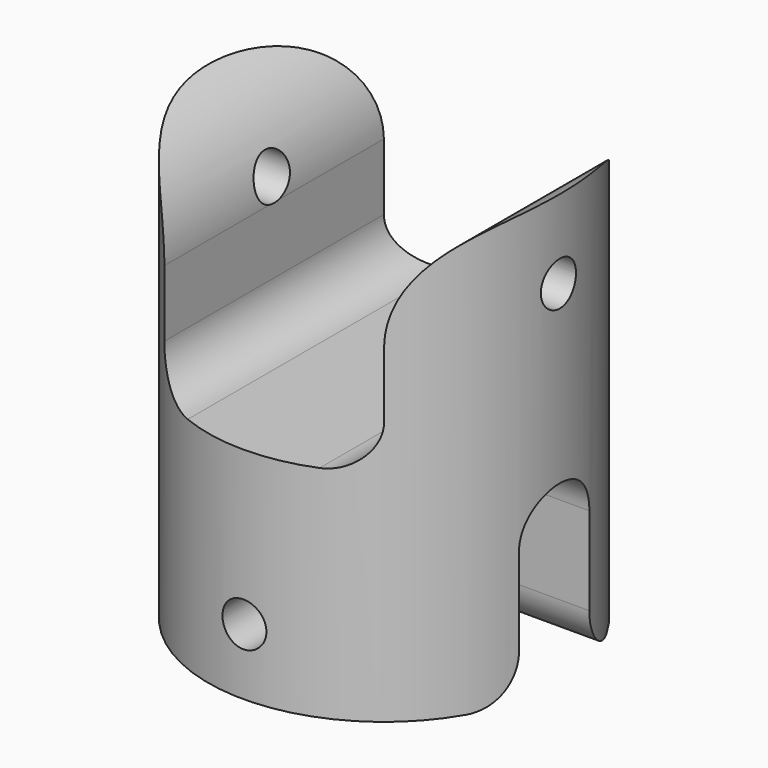
from build123d import *

# Parameters (mm, degrees)
F0_R         = 8
F1_DEPTH     = 20
F3_DEPTH     = 10
F5_DEPTH     = 8
F7_D         = 2
F7_DEPTH     = 3.001
F9_D         = 2
F10_T1_DEPTH = 37.4894960018
F12_D        = 2
F12_DEPTH    = 6.0010001
F14_D        = 2
F15_R        = 2
F16_R        = 1.9999


# Not quite as in the source:
# - a fillet or chamfer that OpenCascade refuses, or shapes differently, is made with other operations: its cross-section is extruded or revolved along the edge and cut away or added
# - a fillet or chamfer is up to 0.001 mm smaller than in the source, because OpenCascade refuses the exact size


with BuildPart() as f1:
    # F0 (on Top) → F1 (new body)
    with BuildSketch(Plane.XY):
        Circle(F0_R)
    extrude(amount=F1_DEPTH)

    # F2 (on face) → F3 (cut)
    with BuildSketch(Plane.XY.offset(20)):
        with BuildLine():
            ThreePointArc((5, 6.2449979984), (0, 8), (-5, 6.2449979984))
            Line((-5, 6.2449979984), (-5, -6.2449979984))
            ThreePointArc((-5, -6.2449979984), (0, -8), (5, -6.2449979984))
            Line((5, -6.2449979984), (5, 6.2449979984))
        make_face()
    extrude(amount=-F3_DEPTH, mode=Mode.SUBTRACT)

    # F4 (on face) → F5 (cut)
    with BuildSketch(Plane.XY):
        with BuildLine():
            ThreePointArc((8, 0), (7.9362375701, 1.0080343399), (7.7459666924, 2))
            Line((7.7459666924, 2), (-7.7459666924, 2))
            ThreePointArc((-7.7459666924, 2), (-7.9362375701, 1.0080343399), (-8, 0))
            ThreePointArc((-8, 0), (-7.9362375701, -1.0080343399), (-7.7459666924, -2))
            Line((-7.7459666924, -2), (7.7459666924, -2))
            ThreePointArc((7.7459666924, -2), (7.9362375701, -1.0080343399), (8, 0))
        make_face()
    extrude(amount=F5_DEPTH, mode=Mode.SUBTRACT)

    # F7 (through all, one way)
    with BuildSketch(Plane.YZ.offset(-5)):
        with Locations((0, 16)):
            Circle(F7_D / 2)
    extrude(amount=-F7_DEPTH, mode=Mode.SUBTRACT)

    # F9 (through all)
    with Locations(Plane(origin=(5, 0, 0), x_dir=(0, -1, 0), z_dir=(-1, 0, 0))):
        with Locations((0, 16)):
            Hole(F9_D / 2)

    # F10: fillet of radius 5 on 2 edges, made by hand

    # F10_s2 → F10_t1 (cut)
    with BuildSketch(Plane.XZ.offset(-18.7447480009)):
        with BuildLine():
            ThreePointArc((9.9999, 20.0001), (6.4643660941, 18.5356339059), (4.9999, 15.0001))
            Line((4.9999, 15.0001), (4.8999, 15.0001))
            ThreePointArc((4.8999, 15.0001), (4.9, 17.50005), (4.9, 20))
            Line((4.9, 20), (5, 20.1))
            ThreePointArc((5, 20.1), (7.49995, 20.1), (9.9999, 20.1001))
            Line((9.9999, 20.1001), (9.9999, 20.0001))
        make_face()
        with BuildLine():
            ThreePointArc((-4.9999, 15.0001), (-6.4643660941, 18.5356339059), (-9.9999, 20.0001))
            Line((-9.9999, 20.0001), (-9.9999, 20.1001))
            ThreePointArc((-9.9999, 20.1001), (-7.49995, 20.1), (-5, 20.1))
            Line((-5, 20.1), (-4.9, 20))
            ThreePointArc((-4.9, 20), (-4.9, 17.50005), (-4.8999, 15.0001))
            Line((-4.8999, 15.0001), (-4.9999, 15.0001))
        make_face()
    extrude(amount=F10_T1_DEPTH, mode=Mode.SUBTRACT)

    # F12 (through all, one way)
    with BuildSketch(Plane(origin=(0, -2, 0), x_dir=(-1, 0, 0), z_dir=(0, 1, 0))):
        with Locations((0, 3)):
            Circle(F12_D / 2)
    extrude(amount=-F12_DEPTH, mode=Mode.SUBTRACT)

    # F14 (through all)
    with Locations(Plane.XZ.offset(-2)):
        with Locations((0, 3)):
            Hole(F14_D / 2)

    # F15
    f15_edges = [f1.edges().sort_by_distance(p)[0] for p in [
        (0, 2, 0),
        (0, -2, 0),
    ]]
    fillet(f15_edges, radius=F15_R)

    # F16 (radius 2 in the source; OpenCascade refuses exactly that, so slightly less here)
    f16_edges = [f1.edges().sort_by_distance(p)[0] for p in [
        (-5, 0, 10),
        (5, 0, 10),
        (0, 2, 8),
        (0, -2, 8),
    ]]
    fillet(f16_edges, radius=F16_R)


solid = f1.part
